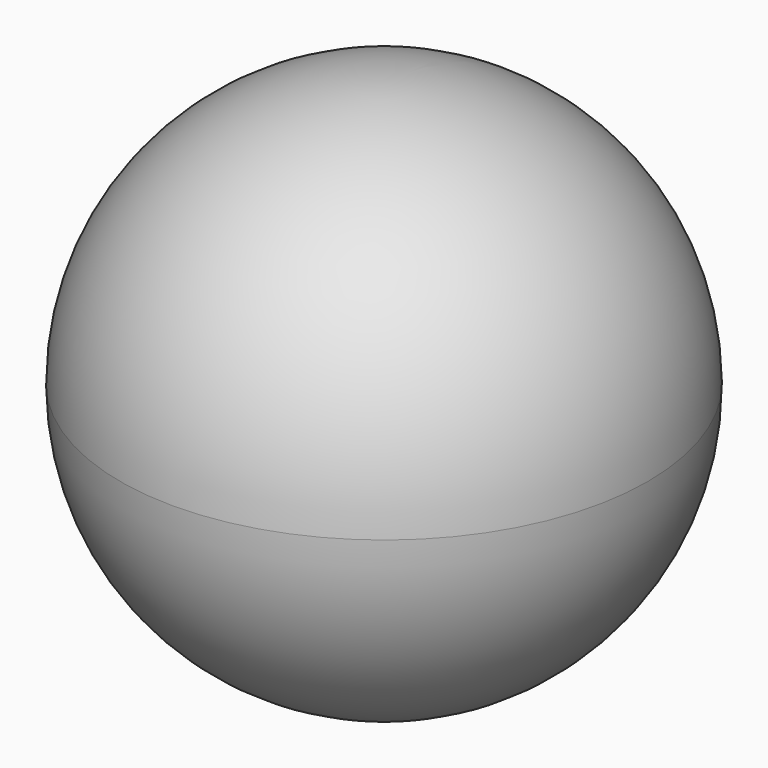
from build123d import *


with BuildPart() as f1:
    # F0 (on Right) → F1 (revolve)
    with BuildSketch(Plane.YZ):
        with BuildLine():
            ThreePointArc((0, -49.0702423129), (34.6979010939, -34.6979010939), (49.0702423129, 0))
            ThreePointArc((49.0702423129, 0), (34.6979010939, 34.6979010939), (0, 49.0702423129))
            Line((0, 49.0702423129), (0, 0))
            Line((0, 0), (0, -49.0702423129))
        make_face()
    revolve(axis=Axis((0, 0, 0), (0, 0, -1)))


solid = f1.part
